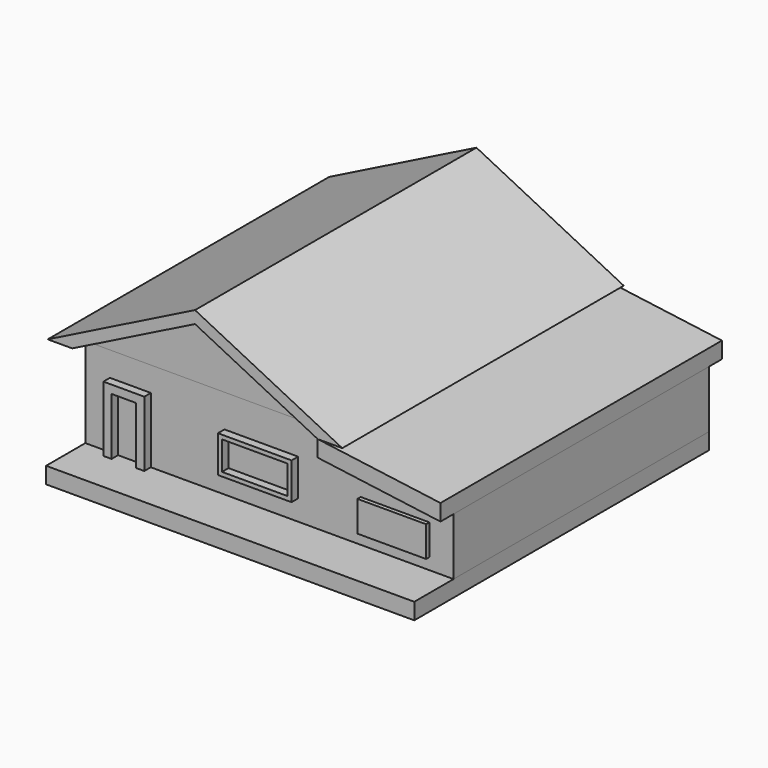
from build123d import *

# Parameters (mm, degrees)
F1_DEPTH      = 914.4
F1_DEPTH_BACK = 12192
F2_DEPTH      = 304.8
F2_DEPTH_BACK = 11582.4
F0_W          = 4572
F0_H          = 609.6
F3_DEPTH      = 2133.6
F3_DEPTH_BACK = 11582.4
F0_W_2        = 2743.2
F0_H_2        = 1371.6
F0_W_3        = 2559.5574378967
F0_H_3        = 1140.672326088
F4_DEPTH      = 304.8
F4_DEPTH_BACK = 11582.4
F0_W_4        = 914.4
F0_H_4        = 2133.6
F5_DEPTH      = 304.8
F0_W_5        = 2438.4
F0_H_5        = 1066.8
F6_DEPTH      = 609.6
F7_W          = 1354.6671867371
F7_H          = 789.4748449326
F8_DEPTH      = 30.48
F7_W_2        = 1802.1693229675
F7_H_2        = 1203.6726474762
F9_DEPTH      = 457.2
F10_DEPTH     = 304.8
F7_W_3        = 1516.5266990662
F7_H_3        = 688.2555484772
F11_DEPTH     = 304.8
F0_W_6        = 1864.025592804
F0_H_6        = 417.3192977905
F13_DEPTH     = 457.2


# Not quite as in the source:
# - the program builds the solid bodies; features that only make, move or delete a surface that nothing else refers to are left out


with BuildPart() as f1:
    # F0 (on Front) → F1 (new body, two sides)
    with BuildSketch(Plane.XZ) as f1_sk:
        Polygon((-5486.4, 0), (-4572, 0), (0, 2286), (0, 2743.2), align=None)
        Polygon((0, 2286), (4572, 0), (5486.4, 0), (0, 2743.2), align=None)
    extrude(amount=F1_DEPTH)
    extrude(f1_sk.sketch, amount=-F1_DEPTH_BACK)



with BuildPart() as f1b:
    # F0 (on Front) → F1, piece 2 (new body, two sides)
    with BuildSketch(Plane.XZ) as f1_2_sk:
        Polygon((9144, -609.6), (4572, 0), (4572, -609.6), (9144, -1219.2), align=None)
    extrude(amount=F1_DEPTH)
    extrude(f1_2_sk.sketch, amount=-F1_DEPTH_BACK)


with BuildPart() as f1_1:
    add(f1.part)

    add(f1b.part)  # F2 merges F1b
    # F0 (on Front) → F2 (join, two sides)
    with BuildSketch(Plane.XZ) as f2_sk:
        Polygon((-4572, 0), (0, 0), (0, 2286), align=None)
        Polygon((0, 2286), (0, 0), (4572, 0), align=None)
    extrude(amount=F2_DEPTH)
    extrude(f2_sk.sketch, amount=-F2_DEPTH_BACK)


with BuildPart() as f3:
    # F0 (on Front) → F3 (new body, two sides)
    with BuildSketch(Plane.XZ) as f3_sk:
        Polygon((-3657.6, -3352.8), (-4572, -3352.8), (-4572, -3962.4), (4572, -3962.4), (4572, -3352.8), (-2133.6, -3352.8), (-2438.4, -3352.8), (-3352.8, -3352.8), align=None)
        with Locations((6858, -3657.6)):
            Rectangle(F0_W, F0_H)
    extrude(amount=F3_DEPTH)
    extrude(f3_sk.sketch, amount=-F3_DEPTH_BACK)

    # F0 (on Front) → F5 (join)
    with BuildSketch(Plane.XZ):
        with Locations((-2895.6, -2286)):
            Rectangle(F0_W_4, F0_H_4)
    extrude(amount=F5_DEPTH)


with BuildPart() as f4:
    # F0 (on Front) → F4 (new body, two sides)
    with BuildSketch(Plane.XZ) as f4_sk:
        Polygon((4572, 0), (0, 0), (-4572, 0), (-4572, -3352.8), (-3657.6, -3352.8), (-3657.6, -914.4), (-2133.6, -914.4), (-2133.6, -3352.8), (4572, -3352.8), (4572, -609.6), align=None)
        with Locations((1981.2, -1905)):
            Rectangle(F0_W_2, F0_H_2, mode=Mode.SUBTRACT)
        Polygon((9144, -1219.2), (4572, -609.6), (4572, -3352.8), (9144, -3352.8), align=None)
        with Locations((6963.0782604218, -2354.5383810997)):
            Rectangle(F0_W_3, F0_H_3, mode=Mode.SUBTRACT)
    extrude(amount=F4_DEPTH)
    extrude(f4_sk.sketch, amount=-F4_DEPTH_BACK)

    # F7 (on face) → F8 (join)
    with BuildSketch(Plane(origin=(-4572, 0, 0), x_dir=(0, -1, 0), z_dir=(-1, 0, 0))):
        with Locations((-7696.8805789948, -1582.2919011116)):
            Rectangle(F7_W, F7_H)
    extrude(amount=F8_DEPTH)

    # F7 (on face) → F9 (join)
    with BuildSketch(Plane(origin=(-4572, 0, 0), x_dir=(0, -1, 0), z_dir=(-1, 0, 0))):
        with Locations((-7672.1346378326, -1597.7395772934)):
            Rectangle(F7_W_2, F7_H_2)
        with Locations((-7696.8805789948, -1582.2919011116)):
            Rectangle(F7_W, F7_H, mode=Mode.SUBTRACT)
    extrude(amount=F9_DEPTH)

    # F10 (add): a face of the model
    f10_faces = [f4.faces().sort_by_distance(p)[0] for p in [
        (-4602.48, 7696.8805789948, -1582.2919011116),
    ]]
    extrude(f10_faces, amount=F10_DEPTH)

    # F7 (on face) → F11 (join)
    with BuildSketch(Plane(origin=(-4572, 0, 0), x_dir=(0, -1, 0), z_dir=(-1, 0, 0))):
        with Locations((-3801.3174533844, -1834.1888189316)):
            Rectangle(F7_W_3, F7_H_3)
    extrude(amount=F11_DEPTH)

    # F0 (on Front) → F13 (join)
    with BuildSketch(Plane.XZ):
        with Locations((6963.0782604218, -2354.5383810997)):
            Rectangle(F0_W_3, F0_H_3)
        with Locations((6976.9885540009, -2382.3595046997)):
            Rectangle(F0_W_6, F0_H_6, mode=Mode.SUBTRACT)
        with Locations((6976.9885540009, -2382.3595046997)):
            Rectangle(F0_W_6, F0_H_6)
    extrude(amount=F13_DEPTH)


with BuildPart() as f5:
    # F0 (on Front) → F5, piece 2 (new body)
    with BuildSketch(Plane.XZ):
        with Locations((1981.2, -1905)):
            Rectangle(F0_W_5, F0_H_5)
    extrude(amount=F5_DEPTH)


with BuildPart() as f6:
    # F0 (on Front) → F6 (new body)
    with BuildSketch(Plane.XZ):
        with Locations((1981.2, -1905)):
            Rectangle(F0_W_2, F0_H_2)
        with Locations((1981.2, -1905)):
            Rectangle(F0_W_5, F0_H_5, mode=Mode.SUBTRACT)
    extrude(amount=F6_DEPTH)


with BuildPart() as f6b:
    # F0 (on Front) → F6, piece 2 (new body)
    with BuildSketch(Plane.XZ):
        Polygon((-3657.6, -914.4), (-3657.6, -3352.8), (-3352.8, -3352.8), (-3352.8, -1219.2), (-2438.4, -1219.2), (-2438.4, -3352.8), (-2133.6, -3352.8), (-2133.6, -914.4), align=None)
    extrude(amount=F6_DEPTH)


solid = Compound([f1_1.part, f3.part, f4.part, f5.part, f6.part, f6b.part])
